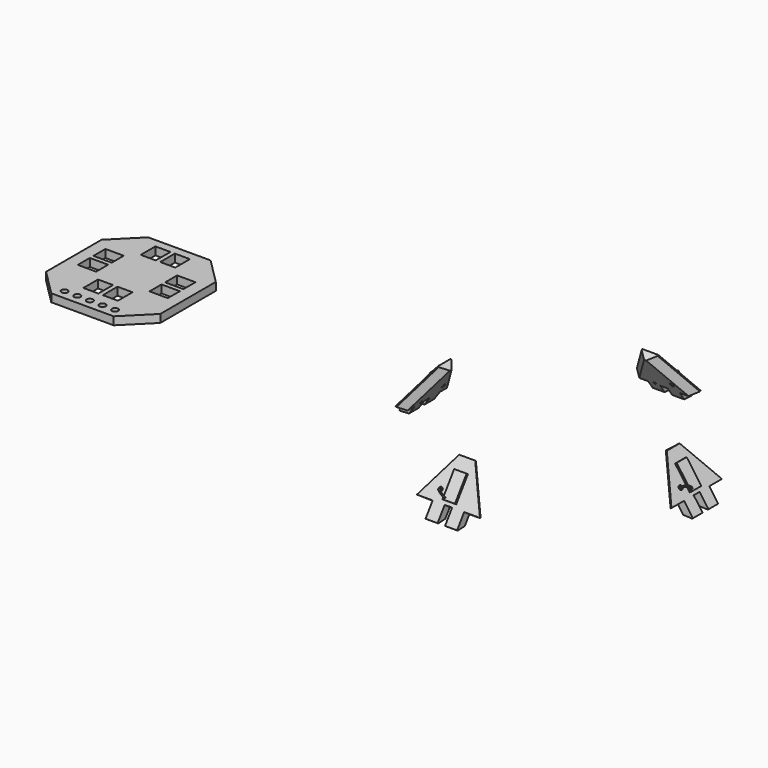
from build123d import *

# Parameters (mm, degrees)
F2_R      = 0.4176776
F2_W      = 0.5
F2_H      = 0.5
F3_DEPTH  = 1.6
F4_DEPTH  = 0.6
F8_DEPTH  = 12.5
F12_R     = 0.125
F13_DEPTH = 0.4
F17_COUNT = 4
F0_R      = 0.635
F18_DEPTH = 1.6


with BuildPart() as f3:
    # F2 (on line) → F3 (new body)
    with BuildSketch(Plane(origin=(0, 0, 0), x_dir=(0, -1, 0), z_dir=(-0.8165408119, 0, 0.5772877121))):
        Polygon((3.175, -2.5537414), (6.3499746, -2.5537414), (1.616583, 5.644769), (-1.616583, 5.644769), (-6.35, -2.5537414), (-3.175, -2.5537414), (-3.175, -5.6447436), (-0.7500112, -5.6447436), (-0.7500112, -2.5537414), (0.7499858, -2.5537414), (0.7499858, -5.6447436), (3.175, -5.6447436), align=None)
        with Locations((-2.5521412, -0.4817872)):
            Circle(F2_R, mode=Mode.SUBTRACT)
        with Locations((1.7124929, -2.3037414)):
            Rectangle(F2_W, F2_H, mode=Mode.SUBTRACT)
        with Locations((1.7124929, -2.3037414)):
            Rectangle(F2_W, F2_H)
    extrude(amount=F3_DEPTH)

    # F2 (on line) → F4 (cut)
    with BuildSketch(Plane(origin=(0, 0, 0), x_dir=(0, -1, 0), z_dir=(-0.8165408119, 0, 0.5772877121))):
        with Locations((1.7124929, -2.3037414)):
            Rectangle(F2_W, F2_H)
    extrude(amount=F4_DEPTH, mode=Mode.SUBTRACT)

    # F7 (on Front) → F8 (cut, symmetric)
    with BuildSketch(Plane.XZ):
        Polygon((-4.4017982548, -3.8009607251), (-3.2586411182, -4.609163522), (-2.6236246349, -3.710968629), align=None)
    extrude(amount=F8_DEPTH, both=True, mode=Mode.SUBTRACT)

    # F10: sweep along a path in F2
    with BuildLine(Plane(origin=(0, 0, 0), x_dir=(0, -1, 0), z_dir=(-0.8165408119, 0, 0.5772877121))) as f10_path:
        Line((-1.616583, 5.644769), (-6.35, -2.5537414))
    # F9 (on face) → F10 (sweep, cut)
    with BuildSketch(Plane(origin=(3.2586557813, 0, 4.6091842622), x_dir=(0.8165408119, 0, -0.5772877121), z_dir=(0.5772877121, 0, 0.8165408119))):
        Polygon((-1.4, 1.616583), (0, 0.216583), (0, 1.616583), align=None)
    sweep(path=f10_path.line, mode=Mode.SUBTRACT)

    # F11: sweep along a path in F2
    with BuildLine(Plane(origin=(0, 0, 0), x_dir=(0, -1, 0), z_dir=(-0.8165408119, 0, 0.5772877121))) as f11_path:
        Line((6.3499746, -2.5537414), (1.616583, 5.644769))
    # F9 (on face) → F11 (sweep, cut)
    with BuildSketch(Plane(origin=(3.2586557813, 0, 4.6091842622), x_dir=(0.8165408119, 0, -0.5772877121), z_dir=(0.5772877121, 0, 0.8165408119))):
        Polygon((-1.4, -1.616583), (0, -1.616583), (0, -0.216583), align=None)
    sweep(path=f11_path.line, mode=Mode.SUBTRACT)

    # F12 (on face) → F13 (join)
    with BuildSketch(Plane(origin=(-1.306465299, 0, 0.9236603393), x_dir=(0, -1, 0), z_dir=(-0.8165408119, 0, 0.5772877121))):
        Polygon((-1.2500127, -1.8552414), (-1.27e-05, -1.8552414), (1.2499873, -1.8552414), (1.2499873, 3.2447586), (-1.2500127, 3.2447586), align=None)
        with Locations((-0.9752485203, -1.5369176399)):
            Circle(F12_R, mode=Mode.SUBTRACT)
        with Locations((-0.9752485203, -1.5369176399)):
            Circle(F12_R)
    extrude(amount=F13_DEPTH)

    # F16: sweep along a path in F15
    with BuildLine(Plane(origin=(-1.0648931339, 1.079330922, -1.2226095381), x_dir=(0.8373088847, 0.3618336096, -0.4098661618), z_dir=(-0.5467301269, 0.554142677, -0.6277038011))) as f16_path:
        add(Plane(origin=(-1.0648931339, 1.079330922, -1.2226095381), x_dir=(0.8373088847, 0.3618336096, -0.4098661618), z_dir=(-0.5467301269, 0.554142677, -0.6277038011)) * Edge.make_bspline(
            [(-1.3481474445, -0.5118566866), (-1.5316580588, -0.5919293312), (-1.8999005009, -0.7725665611), (-2.0950079857, -1.4818432576), (-1.8011752651, -2.1581010096), (-1.3299414377, -2.4063635865), (-0.5833470505, -2.3033206223), (0.0610795409, -1.9937330363), (0.3875084343, -1.8531248746)],
            knots=[0, 0, 0, 0, 0.1525458216, 0.3163655476, 0.4828581917, 0.6211701927, 0.7908775025, 1, 1, 1, 1], degree=3))
    # F12 (on face) → F16 (sweep)
    with BuildSketch(Plane(origin=(-1.306465299, 0, 0.9236603393), x_dir=(0, -1, 0), z_dir=(-0.8165408119, 0, 0.5772877121))):
        with Locations((-0.9752485203, -1.5369176399)):
            Circle(F12_R)
    sweep(path=f16_path.line)


with BuildPart() as f17_1:
    # F17: instance of F3
    add(f3.part.rotate(Axis((25, 0, 13.0700236186), (0, 0, 1)), 1 * 360 / F17_COUNT))


with BuildPart() as f17_2:
    # F17: instance of F3
    add(f3.part.rotate(Axis((25, 0, 13.0700236186), (0, 0, 1)), 2 * 360 / F17_COUNT))


with BuildPart() as f17_3:
    # F17: instance of F3
    add(f3.part.rotate(Axis((25, 0, 13.0700236186), (0, 0, 1)), 3 * 360 / F17_COUNT))


with BuildPart() as f18:
    # F0 (on Top) → F18 (new body)
    with BuildSketch(Plane.XY):
        Polygon((-67.6859915257, -11.8999518454), (-61.3999995257, -11.8999518454), (-55.1140329257, -11.8999518454), (-49.9000479257, -6.6859922454), (-49.9000479257, 7.2839823546), (-55.1160141257, 12.4999485546), (-67.6840103257, 12.4999485546), (-72.8999765257, 7.2839823546), (-72.8999765257, -6.6859922454), align=None)
        with Locations((-66.4799741257, -10.0319596454)):
            Circle(F0_R, mode=Mode.SUBTRACT)
        with Locations((-63.9399741257, -10.0319596454)):
            Circle(F0_R, mode=Mode.SUBTRACT)
        with Locations((-61.3999995257, -10.0319596454)):
            Circle(F0_R, mode=Mode.SUBTRACT)
        with Locations((-58.8599995257, -10.0319596454)):
            Circle(F0_R, mode=Mode.SUBTRACT)
        with Locations((-56.3246731257, -10.0319596454)):
            Circle(F0_R, mode=Mode.SUBTRACT)
        Polygon((-61.8499859257, -3.6409640454), (-61.8499859257, -7.3319650454), (-64.8749735257, -7.3319650454), (-64.8749735257, -7.0319656454), (-64.8749735257, -3.9409634454), (-64.8749735257, -3.6409640454), align=None, mode=Mode.SUBTRACT)
        Polygon((-57.9250001257, -7.3319650454), (-60.9499877257, -7.3319650454), (-60.9499877257, -3.6409640454), (-57.9250001257, -3.6409640454), (-57.9250001257, -3.9409634454), (-57.9250001257, -7.0319656454), align=None, mode=Mode.SUBTRACT)
        Polygon((-70.4659707257, -1.7409678454), (-70.4659707257, 1.2840197546), (-66.7749697257, 1.2840197546), (-66.7749697257, -1.7409678454), (-67.0749691257, -1.7409678454), (-70.1659713257, -1.7409678454), align=None, mode=Mode.SUBTRACT)
        Polygon((-56.0250039257, 1.2840197546), (-52.3340029257, 1.2840197546), (-52.3340029257, -1.7409678454), (-52.6340023257, -1.7409678454), (-55.7250045257, -1.7409678454), (-56.0250039257, -1.7409678454), align=None, mode=Mode.SUBTRACT)
        Polygon((-66.7749697257, 2.1840179546), (-70.4659707257, 2.1840179546), (-70.4659707257, 5.2090055546), (-70.1659713257, 5.2090055546), (-67.0749691257, 5.2090055546), (-66.7749697257, 5.2090055546), align=None, mode=Mode.SUBTRACT)
        Polygon((-52.3340029257, 5.2090055546), (-52.3340029257, 2.1840179546), (-56.0250039257, 2.1840179546), (-56.0250039257, 5.2090055546), (-55.7250045257, 5.2090055546), (-52.6340023257, 5.2090055546), align=None, mode=Mode.SUBTRACT)
        Polygon((-64.8749735257, 10.8000027546), (-61.8499859257, 10.8000027546), (-61.8499859257, 7.1090017546), (-64.8749735257, 7.1090017546), (-64.8749735257, 7.4090011546), (-64.8749735257, 10.5000033546), align=None, mode=Mode.SUBTRACT)
        Polygon((-60.9499877257, 7.1090017546), (-60.9499877257, 10.8000027546), (-57.9250001257, 10.8000027546), (-57.9250001257, 10.5000033546), (-57.9250001257, 7.4090011546), (-57.9250001257, 7.1090017546), align=None, mode=Mode.SUBTRACT)
    extrude(amount=-F18_DEPTH)


solid = Compound([f3.part, f17_1.part, f17_2.part, f17_3.part, f18.part])
